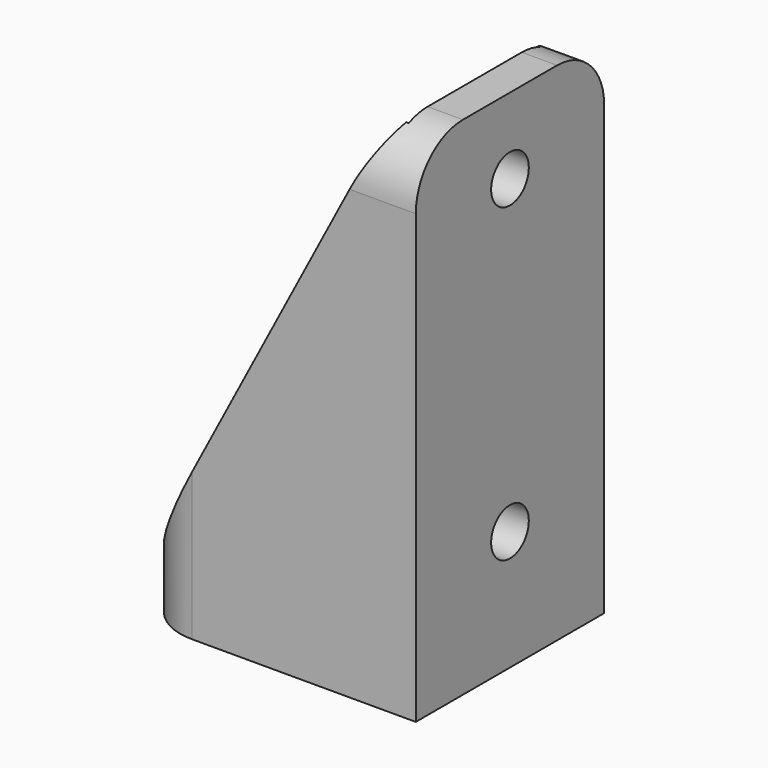
from build123d import *

# Parameters (mm, degrees)
F1_DEPTH        = 3
F2_W            = 3
F2_H            = 20
F3_DEPTH        = 40
F5_DEPTH        = 3
F8_D            = 4
F10_D           = 3.3
F10_CSINK_D     = 7
F10_CSINK_ANGLE = 90
F11_T1_DEPTH    = 28
F11_T3_DEPTH    = 28


# Not quite as in the source:
# - a fillet or chamfer that OpenCascade refuses, or shapes differently, is made with other operations: its cross-section is extruded or revolved along the edge and cut away or added


with BuildPart() as f1:
    # F0 (on Top) → F1 (new body)
    with BuildSketch(Plane.XY):
        Polygon((0, 10), (0, 0), (0, -10), (24, -10), (24, 0), (24, 10), align=None)
    extrude(amount=F1_DEPTH)

    # F2 (on face) → F3 (join)
    with BuildSketch(Plane.XY.offset(3)):
        with Locations((22.5, 0)):
            Rectangle(F2_W, F2_H)
    extrude(amount=F3_DEPTH)

    # F4 (on face) → F5 (join)
    with BuildSketch(Plane.XZ.offset(10)):
        Polygon((21, 3), (21, 43), (0, 3), align=None)
    extrude(amount=-F5_DEPTH)

    # F6: F1 across plane


with BuildPart() as f1_1:
    add(f1.part)
    add(f1.part.mirror(Plane.XZ))

    # F8 (through all)
    with Locations(Plane(origin=(21, 0, 0), x_dir=(0, -1, 0), z_dir=(-1, 0, 0))):
        with Locations((0, 10.16), (0, 36.56)):
            Hole(F8_D / 2)

    # F10 (through all)
    with Locations(Plane.XY.offset(3)):
        with Locations((10.5, 0)):
            CounterSinkHole(F10_D / 2, F10_CSINK_D / 2, counter_sink_angle=F10_CSINK_ANGLE)

    # F11: fillet of radius 5 on 4 edges, made by hand

    # F11_s2 → F11_t1 (cut)
    with BuildSketch(Plane.XY.offset(-12.5)):
        with BuildLine():
            ThreePointArc((0, -5), (1.4644660941, -8.5355339059), (5, -10))
            Line((5, -10), (0, -10))
            Line((0, -10), (0, -5))
        make_face()
        with BuildLine():
            ThreePointArc((0, 5), (1.4644660941, 8.5355339059), (5, 10))
            Line((5, 10), (0, 10))
            Line((0, 10), (0, 5))
        make_face()
    extrude(amount=F11_T1_DEPTH, mode=Mode.SUBTRACT)

    # F11_s4 → F11_t3 (cut)
    with BuildSketch(Plane.YZ.offset(8.5)):
        with BuildLine():
            ThreePointArc((-10, 38), (-8.5355339059, 41.5355339059), (-5, 43))
            Line((-5, 43), (-10, 43))
            Line((-10, 43), (-10, 38))
        make_face()
        with BuildLine():
            ThreePointArc((10, 38), (8.5355339059, 41.5355339059), (5, 43))
            Line((5, 43), (10, 43))
            Line((10, 43), (10, 38))
        make_face()
    extrude(amount=F11_T3_DEPTH, mode=Mode.SUBTRACT)


solid = f1_1.part
